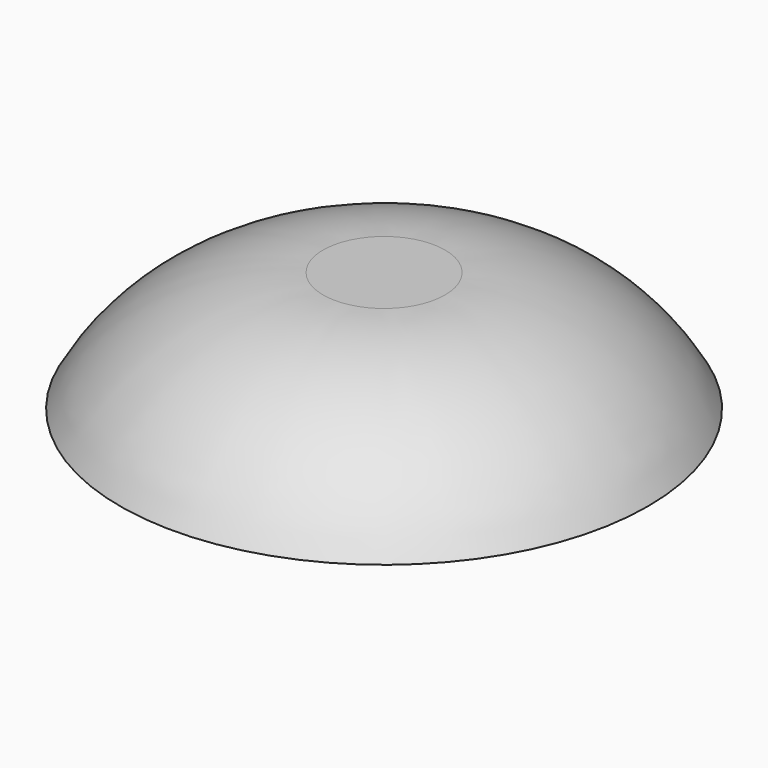
from build123d import *

# Parameters (mm, degrees)
F0_R     = 11
F1_DEPTH = 5
F3_R     = 3.55
F4_DEPTH = 1.5


# Not quite as in the source:
# - a fillet or chamfer that OpenCascade refuses, or shapes differently, is made with other operations: its cross-section is extruded or revolved along the edge and cut away or added


with BuildPart() as f1:
    # F0 (on Top) → F1 (new body)
    with BuildSketch(Plane.XY):
        Circle(F0_R)
    extrude(amount=F1_DEPTH)

    # F2: fillet of radius 9.6568542495 on 1 edges, made by hand

    # F2_s1 → F2_t2 (revolve, cut)
    with BuildSketch(Plane.XZ):
        with BuildLine():
            ThreePointArc((11, 0), (7.4536454326, 3.6565504906), (2.5401807055, 5))
            Line((2.5401807055, 5), (11, 5))
            Line((11, 5), (11, 0))
        make_face()
    revolve(axis=Axis((0, 0, 5), (0, 0, 1)), mode=Mode.SUBTRACT)

    # F3 (on Top) → F4 (cut)
    with BuildSketch(Plane.XY):
        Circle(F3_R)
    extrude(amount=F4_DEPTH, mode=Mode.SUBTRACT)


solid = f1.part
